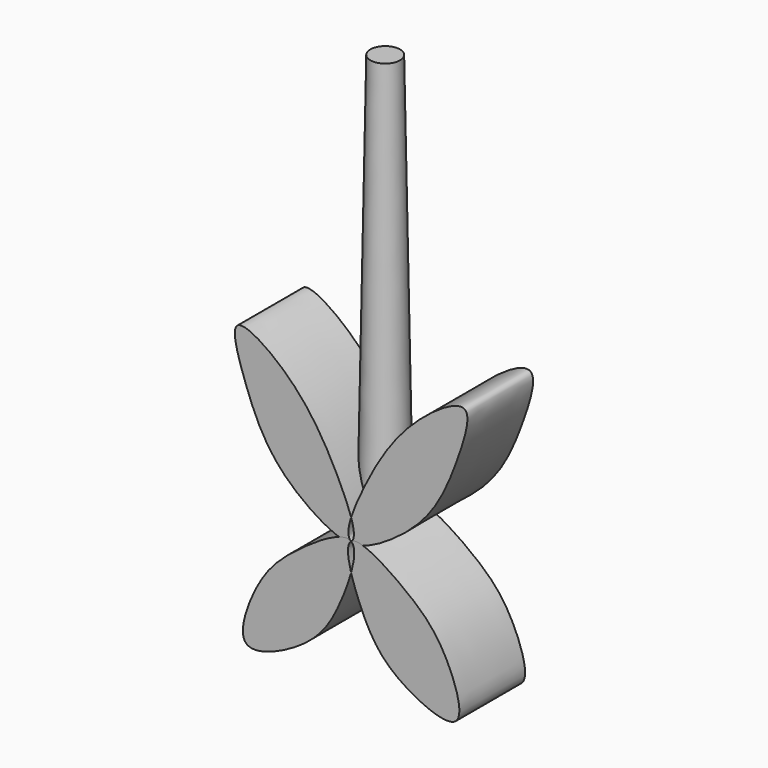
from build123d import *

# Parameters (mm, degrees)
F2_DEPTH = 5.334
F3_R     = 1.427088879
F4_DEPTH = 26.67
F4_TAPER = 1


with BuildPart() as f2:
    # F0 (on Front) → F2 (new body)
    with BuildSketch(Plane.XZ):
        with BuildLine():
            add(Edge.make_bspline(
                [(0, 1.3734232062), (-0.1891456517, 1.9682690903), (-1.3872274811, 4.6479528258), (-3.5359864877, 8.1093093668), (-8.3029516428, 11.1686804607), (-6.7154718992, 6.2014445679), (-4.9282457235, 2.1279215131), (-0.5743113943, -0.4013639182), (0, 0)],
                knots=[0.0787883503, 0.0787883503, 0.0787883503, 0.0787883503, 0.1493641404, 0.34640222, 0.4970269185, 0.6404182512, 0.8287738354, 1, 1, 1, 1], degree=3))
            add(Edge.make_bspline(
                [(0, 0), (-0.2642647953, 0.1846843972), (-0.2111556083, 0.7093580091), (0, 1.3734232062)],
                knots=[0, 0, 0, 0, 0.0787883503, 0.0787883503, 0.0787883503, 0.0787883503], degree=3))
        make_face()
    extrude(amount=F2_DEPTH)


with BuildPart() as f2b:
    # F0 (on Front) → F2, piece 2 (new body)
    with BuildSketch(Plane.XZ):
        with BuildLine():
            add(Edge.make_bspline(
                [(0, 0), (0.2642647953, 0.1846843972), (0.2111556083, 0.7093580091), (0, 1.3734232062)],
                knots=[0, 0, 0, 0, 0.0787883503, 0.0787883503, 0.0787883503, 0.0787883503], degree=3))
            add(Edge.make_bspline(
                [(0, 1.3734232062), (0.1891456517, 1.9682690903), (1.3872274811, 4.6479528258), (3.5359864877, 8.1093093668), (8.3029516428, 11.1686804607), (6.7154718992, 6.2014445679), (4.9282457235, 2.1279215131), (0.5743113943, -0.4013639182), (0, 0)],
                knots=[0.0787883503, 0.0787883503, 0.0787883503, 0.0787883503, 0.1493641404, 0.34640222, 0.4970269185, 0.6404182512, 0.8287738354, 1, 1, 1, 1], degree=3))
        make_face()
    extrude(amount=F2_DEPTH)


with BuildPart() as f2c:
    # F1 (on Front) → F2, piece 3 (new body)
    with BuildSketch(Plane.XZ):
        with BuildLine():
            add(Edge.make_bspline(
                [(0, -1.7959175247), (-0.2337398032, -0.9580135272), (-0.3070084548, -0.234345833), (0, 0)],
                knots=[0.9045673843, 0.9045673843, 0.9045673843, 0.9045673843, 1, 1, 1, 1], degree=3))
            add(Edge.make_bspline(
                [(0, 0), (-0.5336749747, 0.4073650237), (-3.976302372, -1.7841660826), (-6.1917247461, -4.0886252186), (-7.9181121338, -9.2949958308), (-2.5771520257, -6.9829206625), (-1.0584729835, -4.7452005162), (-0.1679340915, -2.3979230226), (0, -1.7959175247)],
                knots=[0, 0, 0, 0, 0.1658911929, 0.3393833044, 0.4969228956, 0.6610761119, 0.8360022986, 0.9045673843, 0.9045673843, 0.9045673843, 0.9045673843], degree=3))
        make_face()
    extrude(amount=F2_DEPTH)


with BuildPart() as f2d:
    # F1 (on Front) → F2, piece 4 (new body)
    with BuildSketch(Plane.XZ):
        with BuildLine():
            add(Edge.make_bspline(
                [(0, 0), (0.5336749747, 0.4073650237), (3.976302372, -1.7841660826), (6.1917247461, -4.0886252186), (7.9181121338, -9.2949958308), (2.5771520257, -6.9829206625), (1.0584729835, -4.7452005162), (0.1679340915, -2.3979230226), (0, -1.7959175247)],
                knots=[0, 0, 0, 0, 0.1658911929, 0.3393833044, 0.4969228956, 0.6610761119, 0.8360022986, 0.9045673843, 0.9045673843, 0.9045673843, 0.9045673843], degree=3))
            add(Edge.make_bspline(
                [(0, -1.7959175247), (0.2337398032, -0.9580135272), (0.3070084548, -0.234345833), (0, 0)],
                knots=[0.9045673843, 0.9045673843, 0.9045673843, 0.9045673843, 1, 1, 1, 1], degree=3))
        make_face()
    extrude(amount=F2_DEPTH)


with BuildPart() as f4:
    # F3 (on Top) → F4 (new body)
    with BuildSketch(Plane.XY):
        with Locations((0, -2.5699601974)):
            Circle(F3_R)
    extrude(amount=F4_DEPTH, taper=F4_TAPER)


solid = Compound([f2.part, f2b.part, f2c.part, f2d.part, f4.part])
